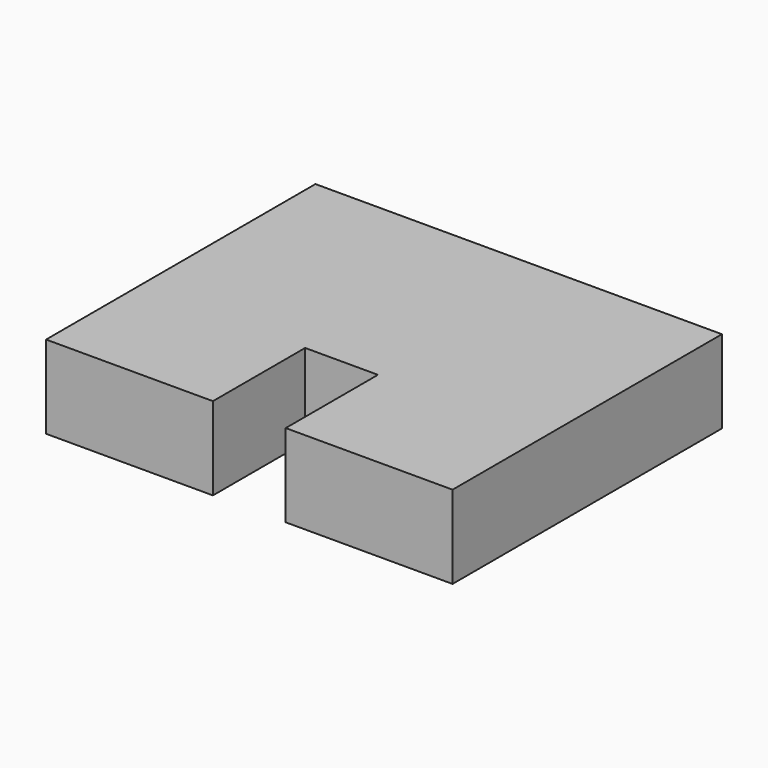
from build123d import *

# Parameters (mm, degrees)
F1_DEPTH = 25.4


# Not quite as in the source:
# - ends of sketch curves that miss each other by under 0.0002 mm in the source are joined


with BuildPart() as f1:
    # F0 (on Top) → F1 (new body)
    with BuildSketch(Plane.XY):
        Polygon((62.2013732791, -51.5250116587), (62.2013732791, 51.5250116587), (-62.2013732791, 51.5250116587), (-62.2013732791, -51.5250116587), (-11.1405421048, -51.5250116587), (-11.1405421048, -16.2466224283), (11.1405421048, -16.2466224283), (11.1405421048, -51.5250060707), align=None)
    extrude(amount=F1_DEPTH)


solid = f1.part
